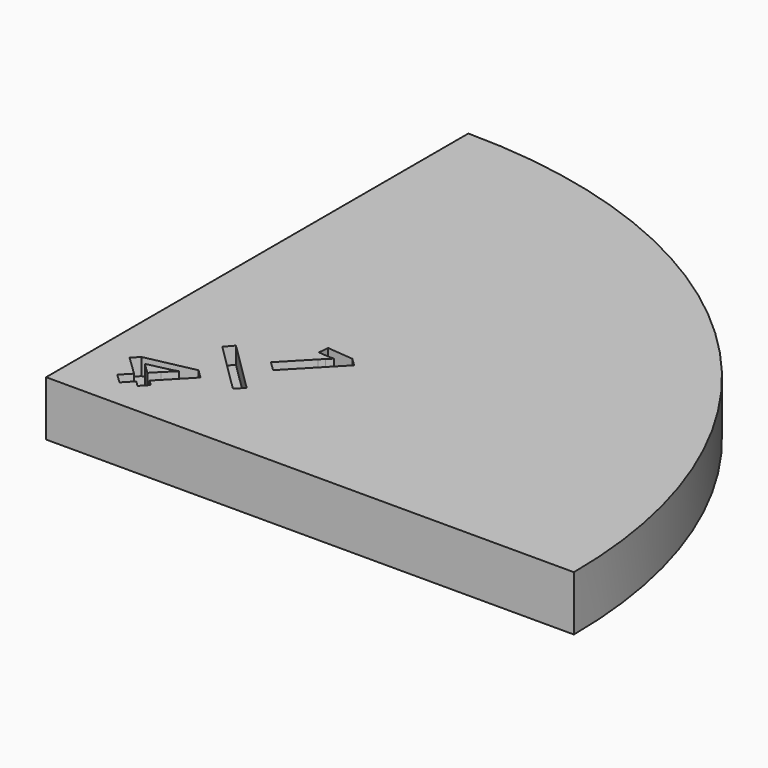
from build123d import *

# Parameters (mm, degrees)
F1_DEPTH     = 6.5
F2_R         = 12.5
F3_DEPTH     = 5
F4_TEXT_SIZE = 10.5901873699
F5_DEPTH     = 2
F7_DEPTH     = 2


# Not quite as in the source:
# - Text() gives the source's letters only with a copy of the font that has no kerning and outlines rounded to 1/6400 em; it was checked with that copy


with BuildPart() as f1:
    # F0 (on Top) → F1 (new body)
    with BuildSketch(Plane.XY):
        with BuildLine():
            Line((0, 0), (62.5, 0))
            ThreePointArc((62.5, 0), (44.1941738242, 44.1941738242), (0, 62.5))
            Line((0, 62.5), (0, 0))
        make_face()
    extrude(amount=F1_DEPTH)

    # F2 (on face) → F3 (cut)
    with BuildSketch(Plane(origin=(0, 0, 0), x_dir=(1, 0, 0), z_dir=(0, 0, -1))):
        with Locations((18.0286169052, -41.4407812059)):
            Circle(F2_R)
        with Locations((40.564391762, -15.9002393484)):
            Circle(F2_R)
    extrude(amount=-F3_DEPTH, mode=Mode.SUBTRACT)

    # F4 (on face) → F5 (cut)
    with BuildSketch(Plane.XY.offset(6.5)):
        with Locations(Location((12.3579710088, 17.2461083728), (0, 0, -43.9134346809))):
            Text('1', F4_TEXT_SIZE, font='Open Sans', font_style=FontStyle.BOLD, text_align=(TextAlign.LEFT, TextAlign.BOTTOM))
        with Locations(Location((2.3687107051, 6.8706014196), (0, 0, -43.9134346809))):
            Text('4', F4_TEXT_SIZE, font='Open Sans', font_style=FontStyle.BOLD, text_align=(TextAlign.LEFT, TextAlign.BOTTOM))
    extrude(amount=-F5_DEPTH, mode=Mode.SUBTRACT)

    # F6 (on face) → F7 (cut)
    with BuildSketch(Plane.XY.offset(6.5)):
        Polygon((15.8243358402, 9.9105084671), (9.757736317, 15.9073778304), (8.9087940219, 14.9394981603), (14.9208641504, 8.9965314249), align=None)
    extrude(amount=-F7_DEPTH, mode=Mode.SUBTRACT)


solid = f1.part
